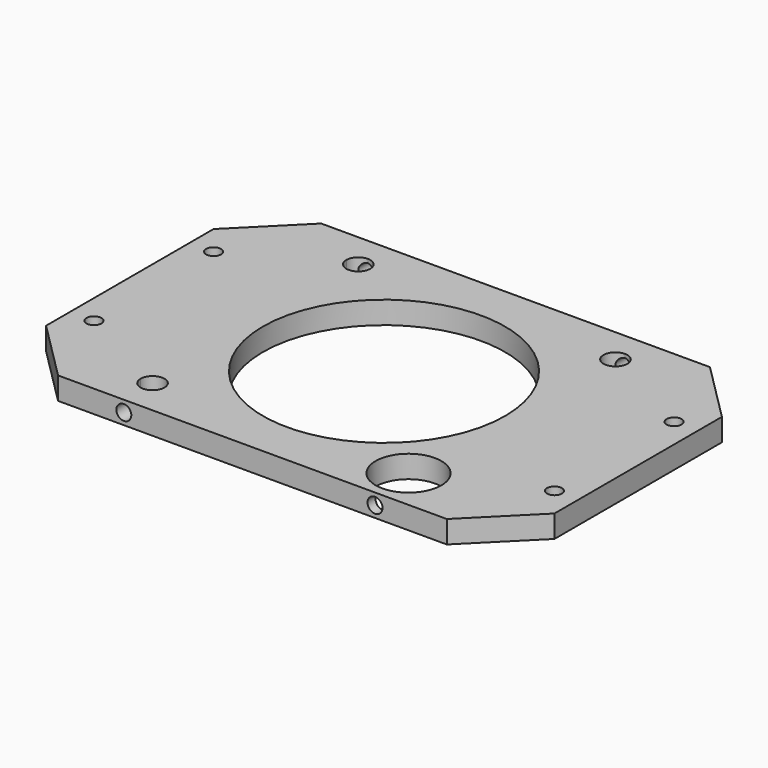
from build123d import *

# Parameters (mm, degrees)
F0_R     = 40.5
F1_DEPTH = 7.5
F3_SIZE  = 20
F2_R     = 2.5
F4_DEPTH = 25
F5_R     = 2.5
F6_DEPTH = 10
F7_R     = 2.5
F8_DEPTH = 10


# Not quite as in the source:
# - a feature names something its author has since deleted; it is built from what else it names


with BuildPart() as f1:
    # F0 (on Top) → F1 (new body)
    with BuildSketch(Plane.XY):
        with BuildLine():
            Line((43, 47), (43, 55))
            Line((43, 55), (-43, 55))
            Line((-43, 55), (-43, 47))
            ThreePointArc((-43, 47), (-40.1715728753, 45.8284271247), (-39, 43))
            ThreePointArc((-39, 43), (-43, 39), (-47, 43))
            Line((-47, 43), (-85, 43))
            Line((-85, 43), (-85, -43))
            Line((-85, -43), (-47, -43))
            ThreePointArc((-47, -43), (-43, -39), (-39, -43))
            ThreePointArc((-39, -43), (-40.1715728753, -45.8284271247), (-43, -47))
            Line((-43, -47), (-43, -55))
            Line((-43, -55), (41, -55))
            Line((41, -55), (85, -55))
            Line((85, -55), (85, 43))
            Line((85, 43), (47, 43))
            ThreePointArc((47, 43), (40.1715728753, 40.1715728753), (43, 47))
        make_face()
        with BuildLine():
            ThreePointArc((52, -41), (48.7781745931, -48.7781745931), (41, -52))
            ThreePointArc((41, -52), (33.2218254069, -33.2218254069), (52, -41))
        make_face(mode=Mode.SUBTRACT)
        Circle(F0_R, mode=Mode.SUBTRACT)
        with BuildLine():
            Line((85, 43), (85, 55))
            Line((85, 55), (43, 55))
            Line((43, 55), (43, 47))
            ThreePointArc((43, 47), (45.8284271247, 45.8284271247), (47, 43))
            Line((47, 43), (85, 43))
        make_face()
        with BuildLine():
            Line((-85, -55), (-43, -55))
            Line((-43, -55), (-43, -47))
            ThreePointArc((-43, -47), (-45.8284271247, -45.8284271247), (-47, -43))
            Line((-47, -43), (-85, -43))
            Line((-85, -43), (-85, -55))
        make_face()
        with BuildLine():
            Line((-43, 47), (-43, 55))
            Line((-43, 55), (-85, 55))
            Line((-85, 55), (-85, 43))
            Line((-85, 43), (-47, 43))
            ThreePointArc((-47, 43), (-45.8284271247, 45.8284271247), (-43, 47))
        make_face()
    extrude(amount=F1_DEPTH)

    # F3
    f3_edges = [f1.edges().sort_by_distance(p)[0] for p in [
        (85, -55, 3.75),
        (-85, -55, 3.75),
        (-85, 55, 3.75),
        (85, 55, 3.75),
    ]]
    chamfer(f3_edges, length=F3_SIZE)

    # F2 (on face) → F4 (cut)
    with BuildSketch(Plane(origin=(0, 0, 0), x_dir=(1, 0, 0), z_dir=(0, 0, -1))):
        with Locations((77, -25)):
            Circle(F2_R)
        with Locations((77, 25)):
            Circle(F2_R)
        with Locations((-77, 25)):
            Circle(F2_R)
        with Locations((-77, -25)):
            Circle(F2_R)
    extrude(amount=-F4_DEPTH, mode=Mode.SUBTRACT)

    # F5 (on face) → F6 (cut)
    with BuildSketch(Plane.XZ.offset(55)):
        with Locations((-43, 3.75)):
            Circle(F5_R)
        with Locations((41, 3.75)):
            Circle(F5_R)
    extrude(amount=-F6_DEPTH, mode=Mode.SUBTRACT)

    # F7 (on face) → F8 (cut)
    with BuildSketch(Plane(origin=(0, 55, 0), x_dir=(-1, 0, 0), z_dir=(0, 1, 0))):
        with Locations((-43, 3.75)):
            Circle(F7_R)
        with Locations((43, 3.75)):
            Circle(F7_R)
    extrude(amount=-F8_DEPTH, mode=Mode.SUBTRACT)


solid = f1.part
